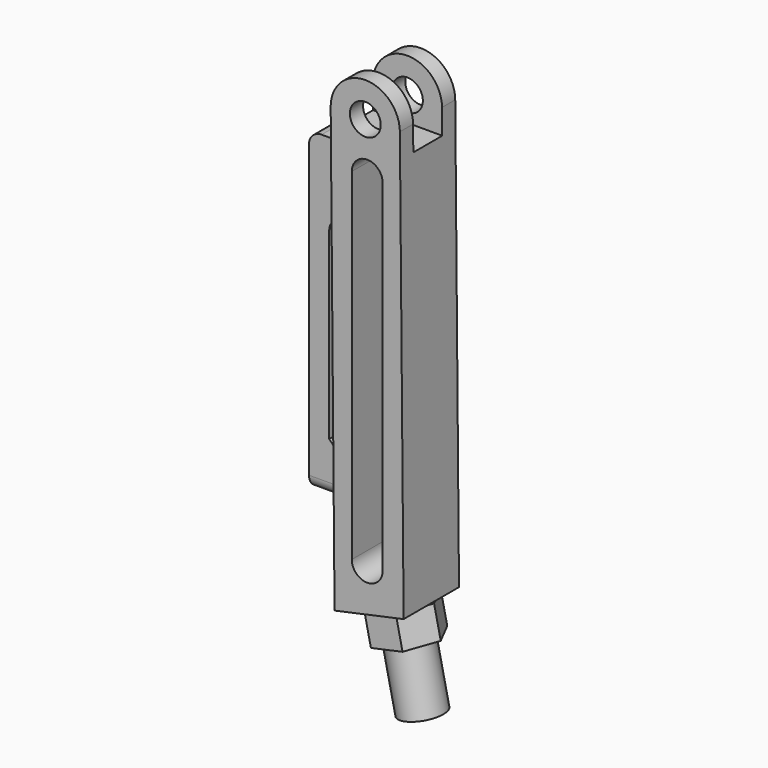
from build123d import *

# Parameters (mm, degrees)
F0_R        = 1.225
F1_DEPTH    = 2.75
F3_DEPTH    = 1.75
F4_W        = 2.8751536738
F4_H        = 5.9757605195
F5_DEPTH    = 13
F6_T1_DEPTH = 3.5
F7_R        = 1
F9_R        = 1.7
F10_DEPTH   = 2.5
F11_DEPTH   = 7.5


# Not quite as in the source:
# - a fillet or chamfer that OpenCascade refuses, or shapes differently, is made with other operations: its cross-section is extruded or revolved along the edge and cut away or added


with BuildPart() as f1:
    # F0 (on Front) → F1 (new body, symmetric)
    with BuildSketch(Plane.XZ):
        with BuildLine():
            Line((-2.7517704794, 0.9889971563), (2.7379837894, 2.1785584332))
            Line((2.7379837894, 2.1785584332), (2.4390654013, 36.1785584332))
            ThreePointArc((2.4390654013, 36.1785584332), (-0.3350046134, 38.9042758715), (-3.0607220517, 36.1302058568))
            Line((-3.0607220517, 36.1302058568), (-2.7517704794, 0.9889971563))
        make_face()
        with BuildLine():
            Line((-1.3813343576, 5.0087761541), (-1.3813707205, 32.1587761541))
            ThreePointArc((-1.3813707205, 32.1587761541), (-0.1563723611, 33.3837777948), (1.0686292795, 32.1587794355))
            Line((1.0686292795, 32.1587794355), (1.0686656424, 5.0087794355))
            ThreePointArc((1.0686656424, 5.0087794355), (-0.1563327169, 3.7837777948), (-1.3813343576, 5.0087761541))
        make_face(mode=Mode.SUBTRACT)
        with Locations((-0.3108283252, 36.154382145)):
            Circle(F0_R, mode=Mode.SUBTRACT)
    extrude(amount=F1_DEPTH, both=True)

    # F2 (on Front) → F3 (join, symmetric)
    with BuildSketch(Plane.XZ):
        Polygon((-2.9082125786, 27.7813646846), (-2.9082125786, 33.2853169523), (-5.5837442831, 33.2853169523), (-5.5837442831, 8.1353169523), (-3.9784252097, 8.1353169523), (-3.9784252097, 12.1868369773), (-3.9784252097, 27.7813646846), align=None)
        with BuildLine():
            Line((-3.9784252097, 12.1868369773), (-3.9784252097, 8.1353169523))
            ThreePointArc((-3.9784252097, 8.1353169523), (-3.0542834819, 10.1610769648), (-3.9784252097, 12.1868369773))
        make_face()
    extrude(amount=F3_DEPTH, both=True)

    # F4 (on Right) → F5 (cut, symmetric)
    with BuildSketch(Plane.YZ):
        with Locations((0, 37.1919497848)):
            Rectangle(F4_W, F4_H)
    extrude(amount=F5_DEPTH, both=True, mode=Mode.SUBTRACT)

    # F6: fillet of radius 1 on 1 edges, made by hand

    # F6_s2 → F6_t1 (join)
    with BuildSketch(Plane.XZ.offset(-1.75)):
        with BuildLine():
            ThreePointArc((-2.9784252097, 27.7813646846), (-3.6855319909, 27.4884714657), (-3.9784252097, 26.7813646846))
            Line((-3.9784252097, 26.7813646846), (-3.9784252097, 27.7813646846))
            Line((-3.9784252097, 27.7813646846), (-2.9784252097, 27.7813646846))
        make_face()
    extrude(amount=F6_T1_DEPTH)

    # F7
    f7_edges = [f1.edges().sort_by_distance(p)[0] for p in [
        (-5.583744, 0, 33.285317),
        (-4.781085, 1.75, 8.135317),
        (-4.781085, -1.75, 8.135317),
    ]]
    fillet(f7_edges, radius=F7_R)

    # F9 (on offset) → F10 (join)
    with BuildSketch(Plane(origin=(-0.3281029821, 0, 1.5141756728), x_dir=(0.9773189207, 0, 0.2117728201), z_dir=(0.2117728201, 0, -0.9773189207))):
        Polygon((2.0697711183, -2.2267070605), (3.3573344565, -0.0034180592), (2.0756913705, 2.2232890013), (-0.4935150537, 2.2267070605), (-1.7810783919, 0.0034180592), (-0.4994353059, -2.2232890013), align=None)
        with Locations((0.7881280323, 0)):
            Circle(F9_R, mode=Mode.SUBTRACT)
    extrude(amount=F10_DEPTH)

    # F11 (add): a face of the model
    f11_faces = [f1.faces().sort_by_distance(p)[0] for p in [
        (0.4421494557, 0, 1.6810797688),
    ]]
    extrude(f11_faces, amount=F11_DEPTH)


solid = f1.part
